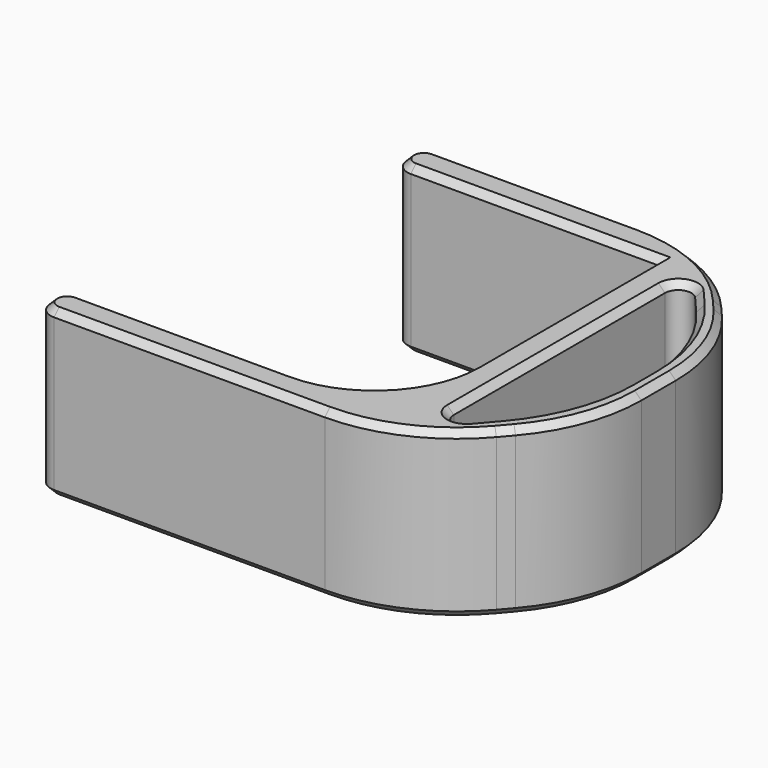
from build123d import *

# Parameters (mm, degrees)
F0_W     = 40
F0_H     = 5
F1_DEPTH = 25
F2_R     = 15
F3_R     = 25
F4_R     = 2.49999
F5_R     = 2
F6_SIZE  = 1


# Not quite as in the source:
# - a fillet or chamfer is up to 0.001 mm smaller than in the source, because OpenCascade refuses the exact size


with BuildPart() as f1:
    # F0 (on Top) → F1 (new body)
    with BuildSketch(Plane.XY):
        Polygon((0, 5), (0, 0), (0, -50), (-50, -50), (-50, -55), (5, -55), (5, -50.3902277714), (5, 0.3902277714), (5, 5), align=None)
        Polygon((20, -12.5), (5, 5), (5, 0.3902277714), (17, -13.6097722286), (17, -36.3902277714), (5, -50.3902277714), (5, -55), (20, -37.5), align=None)
        with Locations((-20, 2.5)):
            Rectangle(F0_W, F0_H)
    extrude(amount=F1_DEPTH)

    # F2
    f2_edges = [f1.edges().sort_by_distance(p)[0] for p in [
        (0, -50, 12.5),
    ]]
    fillet(f2_edges, radius=F2_R)

    # F3
    f3_edges = [f1.edges().sort_by_distance(p)[0] for p in [
        (5, -55, 12.5),
        (20, -37.5, 12.5),
        (20, -12.5, 12.5),
        (5, 5, 12.5),
        (17, -36.390228, 12.5),
        (17, -13.609772, 12.5),
    ]]
    fillet(f3_edges, radius=F3_R)

    # F4 (radius 2.5 in the source; OpenCascade refuses exactly that, so slightly less here)
    f4_edges = [f1.edges().sort_by_distance(p)[0] for p in [
        (-50, -55, 12.5),
        (-50, -50, 12.5),
        (-40, 0, 12.5),
        (-40, 5, 12.5),
    ]]
    fillet(f4_edges, radius=F4_R)

    # F5
    f5_edges = [f1.edges().sort_by_distance(p)[0] for p in [
        (5, -50.390228, 12.5),
        (5, 0.390228, 12.5),
    ]]
    fillet(f5_edges, radius=F5_R)

    # F6
    f6_edges = [f1.edges().sort_by_distance(p)[0] for p in [
        (9.749964, -5.151397, 25),
        (6.306108, -3.140517, 25),
        (15.447125, -14.184218, 25),
        (5, -25, 25),
        (17, -25, 25),
        (6.306108, -46.859483, 25),
        (15.447125, -35.815782, 25),
        (9.749964, -44.848603, 25),
        (-21.999192, 5, 25),
        (-39.26777, 4.26777, 25),
        (3.948047, 2.712822, 25),
        (-40, 2.5, 25),
        (13.232229, -4.604267, 25),
        (-39.26777, 0.73223, 25),
        (18.447125, -13.074446, 25),
        (-18.750005, 0, 25),
        (20, -25, 25),
        (0, -17.5, 25),
        (18.447125, -36.925554, 25),
        (-4.393398, -45.606602, 25),
        (13.232229, -45.395733, 25),
        (-31.250005, -50, 25),
        (3.948047, -52.712822, 25),
        (-49.26777, -50.73223, 25),
        (-26.999192, -55, 25),
        (-50, -52.5, 25),
        (-49.26777, -54.26777, 25),
        (9.749964, -5.151397, 0),
        (6.306108, -3.140517, 0),
        (15.447125, -14.184218, 0),
        (5, -25, 0),
        (17, -25, 0),
        (6.306108, -46.859483, 0),
        (15.447125, -35.815782, 0),
        (9.749964, -44.848603, 0),
        (-21.999192, 5, 0),
        (-39.26777, 4.26777, 0),
        (3.948047, 2.712822, 0),
        (-40, 2.5, 0),
        (13.232229, -4.604267, 0),
        (-39.26777, 0.73223, 0),
        (18.447125, -13.074446, 0),
        (-18.750005, 0, 0),
        (20, -25, 0),
        (0, -17.5, 0),
        (18.447125, -36.925554, 0),
        (-4.393398, -45.606602, 0),
        (13.232229, -45.395733, 0),
        (-31.250005, -50, 0),
        (3.948047, -52.712822, 0),
        (-49.26777, -50.73223, 0),
        (-26.999192, -55, 0),
        (-50, -52.5, 0),
        (-49.26777, -54.26777, 0),
    ]]
    chamfer(f6_edges, length=F6_SIZE)


solid = f1.part
